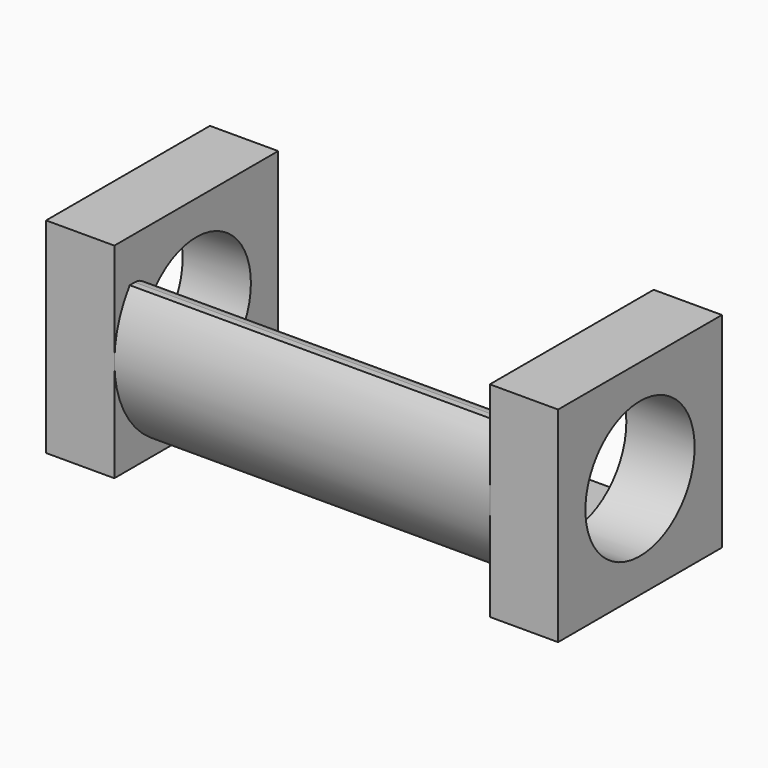
from build123d import *

# Parameters (mm, degrees)
F0_R     = 6
F1_DEPTH = 30
F2_R     = 4
F3_DEPTH = 30.001
F6_DEPTH = 22
F7_W     = 12
F7_H     = 12
F7_R     = 4
F9_DEPTH = 4


# Not quite as in the source:
# - a pattern or mirror of a feature is missing from the dataset's text; its kind, count and spacing are read off the source's solid


with BuildPart() as f1:
    # F0 (on Right) → F1 (new body)
    with BuildSketch(Plane.YZ):
        Circle(F0_R)
    extrude(amount=F1_DEPTH)

    # F2 (on face) → F3 (cut, through all)
    with BuildSketch(Plane.YZ.offset(30)):
        Circle(F2_R)
    extrude(amount=-F3_DEPTH, mode=Mode.SUBTRACT)

    # F5 (on offset) → F6 (cut)
    with BuildSketch(Plane.YZ.offset(26)):
        with BuildLine():
            Line((0, 0), (0, -4))
            Line((0, -4), (8, -4))
            Line((8, -4), (8.9776590466, 9.4645246863))
            Line((8.9776590466, 9.4645246863), (-7.7182371169, 9.4645246863))
            Line((-7.7182371169, 9.4645246863), (-7.7182371169, 3.5))
            Line((-7.7182371169, 3.5), (-4.5, 3.5))
            ThreePointArc((-4.5, 3.5), (-3.7928932188, 3.2071067812), (-3.5, 2.5))
            Line((-3.5, 2.5), (-3.5, 0))
            Line((-3.5, 0), (0, 0))
        make_face()
    extrude(amount=-F6_DEPTH, mode=Mode.SUBTRACT)

    # F7 (on face) → F9 (join)
    with BuildSketch(Plane.YZ.offset(30)):
        Rectangle(F7_W, F7_H)
        Circle(F7_R, mode=Mode.SUBTRACT)
    f9 = extrude(amount=-F9_DEPTH)

    # F9_copies: F9 across plane
    add(f9.mirror(Plane(origin=(15, 0, 0), x_dir=(0, 0, -1), z_dir=(-1, 0, 0))))


solid = f1.part
